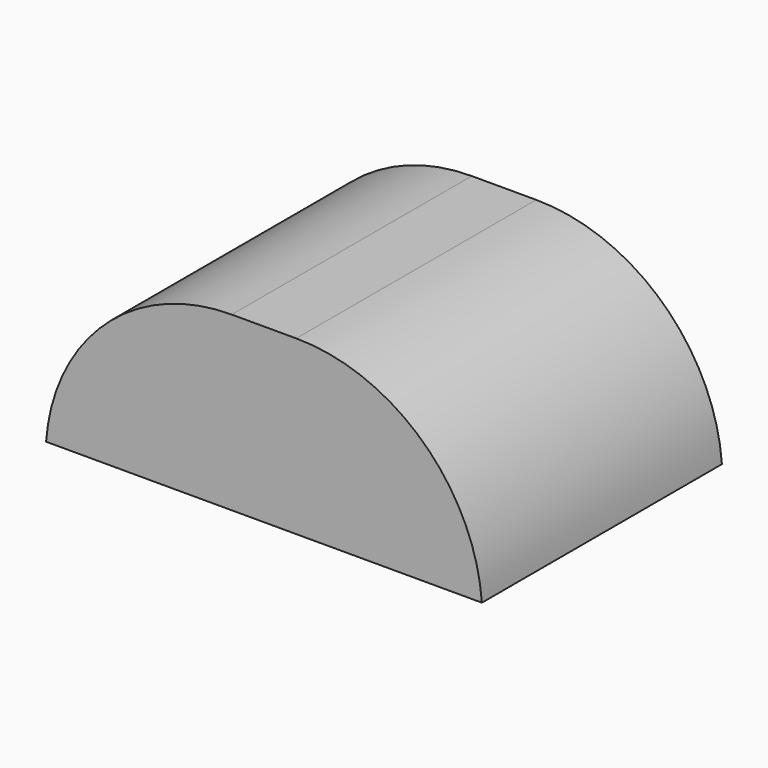
from build123d import *

# Parameters (mm, degrees)
F0_W        = 128.2073557377
F0_H        = 88.262155652
F1_DEPTH    = 50.68946
F2_T1_DEPTH = 361.3524449255
F3_T1_DEPTH = 361.352454187


# Not quite as in the source:
# - a fillet or chamfer that OpenCascade refuses, or shapes differently, is made with other operations: its cross-section is extruded or revolved along the edge and cut away or added


with BuildPart() as f1:
    # F0 (on Top) → F1 (new body)
    with BuildSketch(Plane.XY):
        Rectangle(F0_W, F0_H)
    extrude(amount=F1_DEPTH)

    # F2: fillet of radius 54.7702974041 on 1 edges, made by hand

    # F2_s2 → F2_t1 (cut)
    with BuildSketch(Plane.XZ.offset(-180.6762224627)):
        with BuildLine():
            ThreePointArc((-64.1036778688, 0), (-46.7433494099, 36.0644870809), (-9.4856200142, 50.68946))
            Line((-9.4856200142, 50.68946), (-64.1036778688, 50.68946))
            Line((-64.1036778688, 50.68946), (-64.1036778688, 0))
        make_face()
    extrude(amount=F2_T1_DEPTH, mode=Mode.SUBTRACT)

    # F3: fillet of radius 54.7702994 on 1 edges, made by hand

    # F3_s2 → F3_t1 (cut)
    with BuildSketch(Plane.XZ.offset(-180.6762270935)):
        with BuildLine():
            ThreePointArc((64.1036778688, 0), (46.7433482365, 36.064487178), (9.4856181618, 50.68946))
            Line((9.4856181618, 50.68946), (64.1036778688, 50.68946))
            Line((64.1036778688, 50.68946), (64.1036778688, 0))
        make_face()
    extrude(amount=F3_T1_DEPTH, mode=Mode.SUBTRACT)


solid = f1.part
